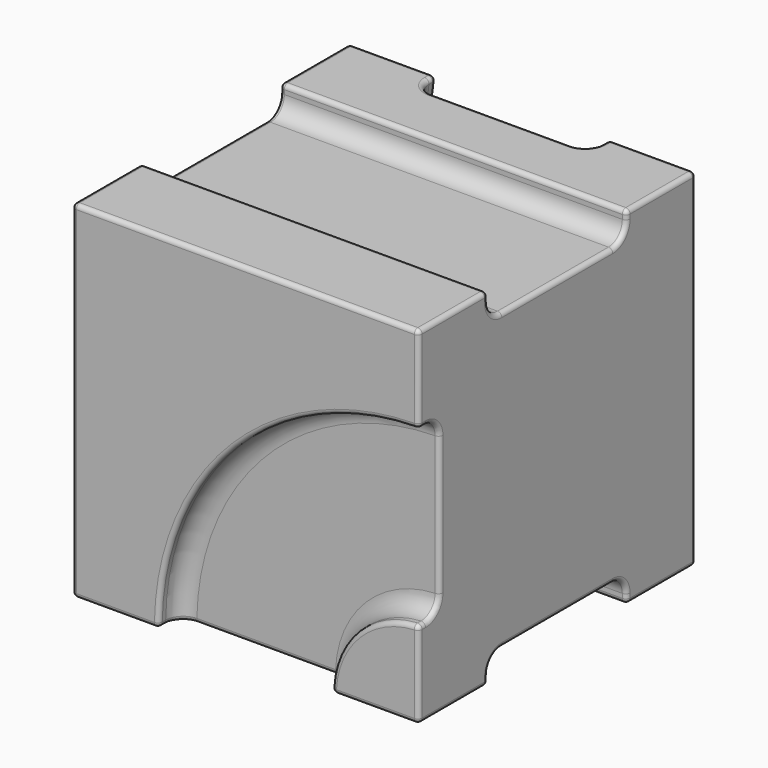
from build123d import *

# Parameters (mm, degrees)
F0_W     = 40
F0_H     = 40
F1_DEPTH = 20
F3_DEPTH = 3
F4_W     = 40
F4_H     = 20
F5_DEPTH = 3
F7_DEPTH = 3
F9_DEPTH = 3
F10_R    = 2
F11_R    = 0.5


# Not quite as in the source:
# - a feature names something its author has since deleted; it is built from what else it names


with BuildPart() as f1:
    # F0 (on Front) → F1 (new body, symmetric)
    with BuildSketch(Plane.XZ):
        Rectangle(F0_W, F0_H)
    extrude(amount=F1_DEPTH, both=True)

    # F2 (on face) → F3 (cut)
    with BuildSketch(Plane.XY.offset(20)):
        Polygon((20, 0), (20, 10), (-20, 10), (-20, 0), (-20, -10), (20, -10), align=None)
    extrude(amount=-F3_DEPTH, mode=Mode.SUBTRACT)

    # F4 (on face) → F5 (cut)
    with BuildSketch(Plane(origin=(0, 0, -20), x_dir=(1, 0, 0), z_dir=(0, 0, -1))):
        Rectangle(F4_W, F4_H)
    extrude(amount=-F5_DEPTH, mode=Mode.SUBTRACT)

    # F6 (on face) → F7 (cut)
    with BuildSketch(Plane.XZ.offset(20)):
        with BuildLine():
            Line((-10, -20), (10, -20))
            ThreePointArc((10, -20), (12.9289321881, -12.9289321881), (20, -10))
            Line((20, -10), (20, 10))
            ThreePointArc((20, 10), (-1.2132034356, 1.2132034356), (-10, -20))
        make_face()
    extrude(amount=-F7_DEPTH, mode=Mode.SUBTRACT)

    # F8 (on face) → F9 (cut)
    with BuildSketch(Plane(origin=(0, 20, 0), x_dir=(-1, 0, 0), z_dir=(0, 1, 0))):
        with BuildLine():
            Line((20, -10), (20, 10))
            ThreePointArc((20, 10), (12.9289321881, 12.9289321881), (10, 20))
            Line((10, 20), (-10, 20))
            ThreePointArc((-10, 20), (-1.2132034356, -1.2132034356), (20, -10))
        make_face()
    extrude(amount=-F9_DEPTH, mode=Mode.SUBTRACT)

    # F10
    f10_edges = [f1.edges().sort_by_distance(p)[0] for p in [
        (0, 10, -17),
        (0, -10, -17),
        (-1.213203, -17, 1.213203),
        (12.928932, -17, -12.928932),
        (-12.928932, 17, 12.928932),
        (0, -10, 17),
        (0, 10, 17),
        (1.213203, 17, -1.213203),
    ]]
    fillet(f10_edges, radius=F10_R)

    # F11
    f11_edges = [f1.edges().sort_by_distance(p)[0] for p in [
        (-20, -20, 0),
        (0, -20, 20),
        (20, -20, 15),
        (-1.213203, -20, 1.213203),
        (-15, -20, -20),
        (12.928932, -20, -12.928932),
        (20, -20, -15),
        (15, -20, -20),
        (-20, 10, 19.5),
        (-20, 9.414214, 17.585786),
        (-20, 15, 20),
        (-20, 0, 17),
        (-20, 20, 15),
        (-20, -9.414214, 17.585786),
        (-20, 19.5, 10),
        (-20, -10, 19.5),
        (-20, 17.585786, 9.414214),
        (-20, -15, 20),
        (-20, 17, 0),
        (-20, 17.585786, -9.414214),
        (-20, -15, -20),
        (-20, 19.5, -10),
        (-20, -10, -19.5),
        (-20, 20, -15),
        (-20, -9.414214, -17.585786),
        (-20, 15, -20),
        (-20, 0, -17),
        (-20, 10, -19.5),
        (-20, 9.414214, -17.585786),
        (-10, -19.5, -20),
        (-9.414214, -17.585786, -20),
        (0, -17, -20),
        (9.414214, -17.585786, -20),
        (0, -10, -20),
        (10, -19.5, -20),
        (20, -15, -20),
        (0, 10, -20),
        (20, 15, -20),
        (0, 20, -20),
        (-15, 20, 20),
        (-12.928932, 20, 12.928932),
        (1.213203, 20, -1.213203),
        (15, 20, 20),
        (20, 20, 0),
        (20, 10, -19.5),
        (20, 9.414214, -17.585786),
        (20, 0, -17),
        (20, -9.414214, -17.585786),
        (20, 15, 20),
        (20, -10, -19.5),
        (20, 10, 19.5),
        (20, 9.414214, 17.585786),
        (20, 0, 17),
        (20, -19.5, -10),
        (20, -9.414214, 17.585786),
        (20, -17.585786, -9.414214),
        (20, -10, 19.5),
        (20, -17, 0),
        (20, -15, 20),
        (20, -17.585786, 9.414214),
        (20, -19.5, 10),
        (-10, 19.5, 20),
        (-9.414214, 17.585786, 20),
        (0, 17, 20),
        (9.414214, 17.585786, 20),
        (0, 10, 20),
        (10, 19.5, 20),
        (0, -10, 20),
    ]]
    fillet(f11_edges, radius=F11_R)


solid = f1.part
